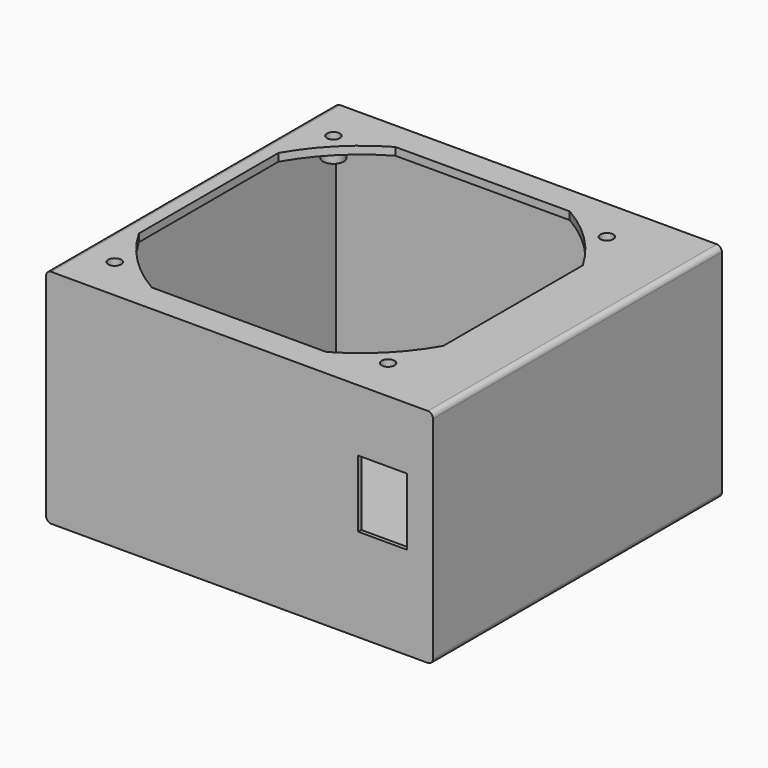
from build123d import *

# Parameters (mm, degrees)
F0_W     = 150
F0_H     = 140
F1_DEPTH = 86
F3_DEPTH = 3
F2_R     = 2.5
F4_DEPTH = 6
F5_T     = -1.5
F6_W     = 19
F6_H     = 26
F7_DEPTH = 10
F8_R     = 10
F9_DEPTH = 5
F10_R    = 2


# Not quite as in the source:
# - a shell that OpenCascade refuses in one call is made with other operations: the cavity is built on its own and cut out


with BuildPart() as f1:
    # F0 (on Top) → F1 (new body)
    with BuildSketch(Plane.XY):
        Rectangle(F0_W, F0_H)
    extrude(amount=F1_DEPTH)

    # F2 (on face) → F3 (cut)
    with BuildSketch(Plane.XY.offset(86)):
        with BuildLine():
            Line((24.8082830088, 59), (-42.8082830088, 59))
            ThreePointArc((-42.8082830088, 59), (-57.0832611207, 48.0832611207), (-68, 33.8082830088))
            Line((-68, 33.8082830088), (-68, -33.8082830088))
            ThreePointArc((-68, -33.8082830088), (-57.0832611207, -48.0832611207), (-42.8082830088, -59))
            Line((-42.8082830088, -59), (24.8082830088, -59))
            ThreePointArc((24.8082830088, -59), (39.0832611207, -48.0832611207), (50, -33.8082830088))
            Line((50, -33.8082830088), (50, 33.8082830088))
            ThreePointArc((50, 33.8082830088), (39.0832611207, 48.0832611207), (24.8082830088, 59))
        make_face()
    extrude(amount=-F3_DEPTH, mode=Mode.SUBTRACT)

    # F2 (on face) → F4 (cut)
    with BuildSketch(Plane.XY.offset(86)):
        with Locations((-62, 53)):
            Circle(F2_R)
        with Locations((44, 53)):
            Circle(F2_R)
        with Locations((44, -53)):
            Circle(F2_R)
        with Locations((-62, -53)):
            Circle(F2_R)
    extrude(amount=-F4_DEPTH, mode=Mode.SUBTRACT)

    # F5: a shell. OpenCascade refuses it in one call, so the cavity is built on its own and cut out:
    # the body offset inwards by the wall thickness, plus a prism from it out through each open face.
    f5_core = offset(f1.part, amount=F5_T, kind=Kind.INTERSECTION, mode=Mode.PRIVATE)
    f5_exits = [f5_core.faces().sort_by_distance(p)[0] for p in [
        (-9, 0, 81.5),
    ]]
    add(f5_core, mode=Mode.SUBTRACT)
    extrude(f5_exits, amount=-F5_T, mode=Mode.SUBTRACT)

    # F6 (on face) → F7 (cut)
    with BuildSketch(Plane.XZ.offset(70)):
        with Locations((55.5, 49)):
            Rectangle(F6_W, F6_H)
    extrude(amount=-F7_DEPTH, mode=Mode.SUBTRACT)

    # F8 (on face) → F9 (cut)
    with BuildSketch(Plane(origin=(0, 70, 0), x_dir=(-1, 0, 0), z_dir=(0, 1, 0))):
        with Locations((-64, 56)):
            Circle(F8_R)
    extrude(amount=-F9_DEPTH, mode=Mode.SUBTRACT)

    # F10
    f10_edges = [f1.edges().sort_by_distance(p)[0] for p in [
        (75, 0, 86),
        (75, 0, 0),
        (-75, 0, 86),
        (-75, 0, 0),
    ]]
    fillet(f10_edges, radius=F10_R)


solid = f1.part
